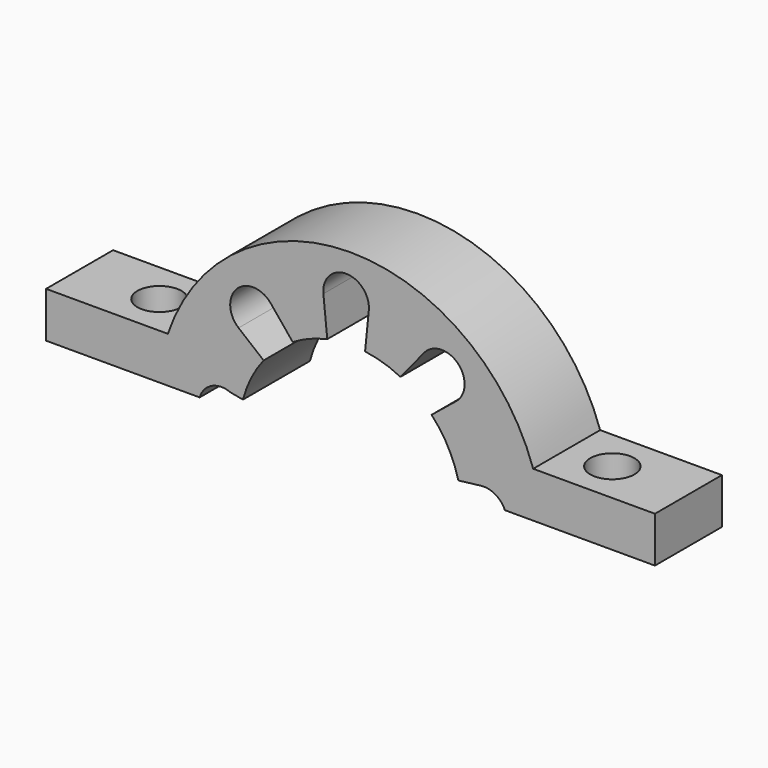
from build123d import *

# Parameters (mm, degrees)
F1_DEPTH = 5.5
F2_R     = 1.45
F3_DEPTH = 25
F4_R     = 1.45
F5_DEPTH = 25


# Not quite as in the source:
# - a feature names something its author has since deleted; it is built from what else it names


with BuildPart() as f1:
    # F0 (on Front) → F1 (new body)
    with BuildSketch(Plane.XZ):
        with BuildLine():
            Line((10.1409122915, -7.7475719752), (20, -7.7475719752))
            Line((20, -7.7475719752), (20, -4.7475719752))
            Line((20, -4.7475719752), (12, -4.7475719752))
            ThreePointArc((12, -4.7475719752), (0, 3.8721859892), (-12, -4.7475719752))
            Line((-12, -4.7475719752), (-20, -4.7475719752))
            Line((-20, -4.7475719752), (-20, -7.7475719752))
            Line((-20, -7.7475719752), (-10, -7.7475719752))
            Line((-10, -7.7475719752), (-9.9101597832, -7.7475719752))
            ThreePointArc((-9.9101597832, -7.7475719752), (-9.399666092, -6.9954026392), (-8.5485111922, -6.6761882044))
            ThreePointArc((-8.5485111922, -6.6761882044), (-8.20089019, -6.698967849), (-7.8678987383, -6.8013200176))
            Line((-7.8678987383, -6.8013200176), (-7.0639233089, -6.9491323338))
            ThreePointArc((-7.0639233089, -6.9491323338), (-6.5280807154, -5.5234621099), (-5.7080769948, -4.2400070969))
            Line((-5.7080769948, -4.2400070969), (-7.3540770708, -2.8946497535))
            ThreePointArc((-7.3540770708, -2.8946497535), (-7.4654597138, -0.6725800185), (-5.2433899789, -0.7839626615))
            Line((-5.2433899789, -0.7839626615), (-3.7957894574, -2.5550538739))
            ThreePointArc((-3.7957894574, -2.5550538739), (-2.6997185699, -2.0081537307), (-1.5276324855, -1.6522248506))
            Line((-1.5276324855, -1.6522248506), (-1.7831469906, 0.8901123752))
            ThreePointArc((-1.7831469906, 0.8901123752), (-0.2906658349, 2.5401123752), (1.2018153207, 0.8901123752))
            Line((1.2018153207, 0.8901123752), (0.9562236033, -1.55349436))
            ThreePointArc((0.9562236033, -1.55349436), (2.1490849475, -1.8141042253), (3.281823707, -2.2698877168))
            Line((3.281823707, -2.2698877168), (4.832326413, -0.3728990956))
            ThreePointArc((4.832326413, -0.3728990956), (7.0560350494, -0.2631578905), (6.9394170389, -2.4865164921))
            Line((6.9394170389, -2.4865164921), (5.9372443956, -3.3004847472))
            Line((5.9372443956, -3.3004847472), (5.3253136848, -3.7974970895))
            ThreePointArc((5.3253136848, -3.7974970895), (6.4103242472, -5.2980690002), (7.0828602188, -7.0233687847))
            Line((7.0828602188, -7.0233687847), (8.5816167977, -6.8438853729))
            ThreePointArc((8.5816167977, -6.8438853729), (9.5121128892, -7.0354424826), (10.1409122915, -7.7475719752))
        make_face()
    extrude(amount=F1_DEPTH)

    # F2 (on face) → F3 (cut)
    with BuildSketch(Plane.XY.offset(-4.7475719752)):
        with Locations((-14.75, -2.75)):
            Circle(F2_R)
    extrude(amount=-F3_DEPTH, mode=Mode.SUBTRACT)

    # F4 (on face) → F5 (cut)
    with BuildSketch(Plane.XY.offset(-4.7475719752)):
        with Locations((15, -2.75)):
            Circle(F4_R)
    extrude(amount=-F5_DEPTH, mode=Mode.SUBTRACT)


solid = f1.part
